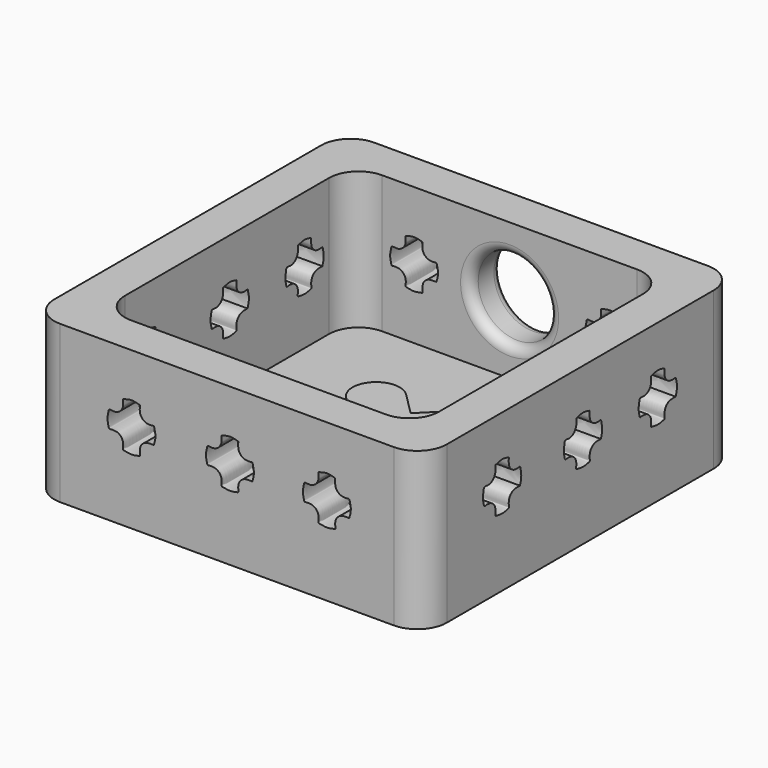
from build123d import *

# Parameters (mm, degrees)
F1_DEPTH      = 2
F2_W          = 40
F2_H          = 40
F3_DEPTH      = 2
F3_DEPTH_BACK = 14
F4_DEPTH      = 2
F5_R          = 3
F6_R          = 4
F7_DEPTH      = 25
F8_R          = 1
F10_DEPTH     = 25
F12_DEPTH     = 45.8


# Not quite as in the source:
# - a pattern or mirror of a feature is missing from the dataset's text; its kind, count and spacing are read off the source's solid


with BuildPart() as f1:
    # F0 (on Top) → F1 (new body)
    with BuildSketch(Plane.XY):
        with BuildLine():
            Line((4, -0.6058874503), (1.6970562748, 1.6970562748))
            ThreePointArc((1.6970562748, 1.6970562748), (-1.6970562748, 1.6970562748), (-1.6970562748, -1.6970562748))
            Line((-1.6970562748, -1.6970562748), (0.6058874503, -4))
            Line((0.6058874503, -4), (-1.6970562748, -6.3029437252))
            ThreePointArc((-1.6970562748, -6.3029437252), (-1.6970562748, -9.6970562748), (1.6970562748, -9.6970562748))
            Line((1.6970562748, -9.6970562748), (4, -7.3941125497))
            Line((4, -7.3941125497), (6.3029437252, -9.6970562748))
            ThreePointArc((6.3029437252, -9.6970562748), (9.6970562748, -9.6970562748), (9.6970562748, -6.3029437252))
            Line((9.6970562748, -6.3029437252), (7.3941125497, -4))
            Line((7.3941125497, -4), (9.6970562748, -1.6970562748))
            ThreePointArc((9.6970562748, -1.6970562748), (9.6970562748, 1.6970562748), (6.3029437252, 1.6970562748))
            Line((6.3029437252, 1.6970562748), (4, -0.6058874503))
        make_face()
    extrude(amount=F1_DEPTH)

    # F2 (on Top) → F4 (join)
    with BuildSketch(Plane.XY):
        with BuildLine():
            Line((17, 12), (-9, 12))
            ThreePointArc((-9, 12), (-11.1213203436, 11.1213203436), (-12, 9))
            Line((-12, 9), (-12, -17))
            ThreePointArc((-12, -17), (-11.1213203436, -19.1213203436), (-9, -20))
            Line((-9, -20), (17, -20))
            ThreePointArc((17, -20), (19.1213203436, -19.1213203436), (20, -17))
            Line((20, -17), (20, 9))
            ThreePointArc((20, 9), (19.1213203436, 11.1213203436), (17, 12))
        make_face()
    extrude(amount=-F4_DEPTH)


with BuildPart() as f3:
    # F2 (on Top) → F3 (new body, two sides)
    with BuildSketch(Plane.XY) as f3_sk:
        with Locations((4, -4)):
            Rectangle(F2_W, F2_H)
        with BuildLine():
            ThreePointArc((-12, 9), (-11.1213203436, 11.1213203436), (-9, 12))
            Line((-9, 12), (17, 12))
            ThreePointArc((17, 12), (19.1213203436, 11.1213203436), (20, 9))
            Line((20, 9), (20, -17))
            ThreePointArc((20, -17), (19.1213203436, -19.1213203436), (17, -20))
            Line((17, -20), (-9, -20))
            ThreePointArc((-9, -20), (-11.1213203436, -19.1213203436), (-12, -17))
            Line((-12, -17), (-12, 9))
        make_face(mode=Mode.SUBTRACT)
    extrude(amount=-F3_DEPTH)
    extrude(f3_sk.sketch, amount=F3_DEPTH_BACK)

    # F5
    f5_edges = [f3.edges().sort_by_distance(p)[0] for p in [
        (-16, -24, 6),
        (-16, 16, 6),
        (24, 16, 6),
        (24, -24, 6),
    ]]
    fillet(f5_edges, radius=F5_R)

    # F6 (on face) → F7 (cut)
    with BuildSketch(Plane(origin=(0, 16, 0), x_dir=(-1, 0, 0), z_dir=(0, 1, 0))):
        with Locations((-4, 7)):
            Circle(F6_R)
    extrude(amount=-F7_DEPTH, mode=Mode.SUBTRACT)

    # F8
    f8_edges = [f3.edges().sort_by_distance(p)[0] for p in [
        (8, 16, 7),
        (8, 12, 7),
    ]]
    fillet(f8_edges, radius=F8_R)

    # F9 (on face) → F10 (cut)
    with BuildSketch(Plane.XZ.offset(24)):
        with BuildLine():
            add(Edge.make_bspline(
                [(-6.5840265518, 9.3437267381), (-6.286408434, 9.4275877117), (-5.7023076012, 9.5950066295), (-5.1532978898, 9.4254739497), (-4.8840257185, 9.3437267381)],
                knots=[0, 0, 0, 0, 0.5095712537, 1, 1, 1, 1], degree=3))
            add(Edge.make_bspline(
                [(-6.5840265518, 9.3437267381), (-6.5841696509, 9.2446224959), (-6.5844438767, 9.0547054322), (-6.5825932662, 8.7979336724), (-6.5988182275, 8.609172852), (-6.7707458313, 8.2509387062), (-6.9735726246, 8.079923012), (-7.250701533, 7.9446481243), (-7.5437717101, 7.8925599497), (-8.077660269, 8.0248628406), (-8.0810784131, 7.6236458981), (-8.1649065579, 7.3625472686), (-8.1781814391, 7.0265606699), (-8.1535417531, 6.7364119598), (-8.0802507294, 6.4930721252), (-8.0454514039, 6.1628262916), (-7.7981073276, 6.2405421407), (-7.4978512443, 6.2260779569), (-7.2459325913, 6.194091152), (-7.0561037114, 6.118114005), (-6.8276872429, 5.9377813233), (-6.7252267328, 5.7961916646), (-6.6269718231, 5.6163632202), (-6.5808026719, 5.3578690355), (-6.5679532623, 5.1331167152), (-6.6600281407, 4.7409543997), (-6.3080518593, 4.7336285908), (-5.9846905263, 4.6481815982), (-5.698126367, 4.6467208848), (-5.4347625835, 4.6517875366), (-5.0847116703, 4.7519672139), (-4.8238785102, 4.7525241561), (-4.8965607786, 5.139699186), (-4.8941701444, 5.3873990167), (-4.7921945694, 5.737853877), (-4.6502771673, 5.9263389013), (-4.3801585127, 6.1591111569), (-3.953865455, 6.2407381261), (-3.6306534992, 6.2287716349), (-3.4628957185, 6.222560627)],
                knots=[0, 0, 0, 0, 0.0273605905, 0.0524320947, 0.0745076412, 0.1056108167, 0.1318649214, 0.158948127, 0.1874687016, 0.220995097, 0.2482860623, 0.2755720453, 0.3045111481, 0.3315301836, 0.3578655515, 0.3837385363, 0.4059679792, 0.434252013, 0.4594532962, 0.4822711791, 0.5090972104, 0.530231005, 0.5527300135, 0.5781274322, 0.6031996615, 0.6315546276, 0.6576667534, 0.6876672756, 0.714256594, 0.7402463844, 0.7710533559, 0.7932728015, 0.8216277676, 0.8482190477, 0.8777914221, 0.9023565188, 0.9315770045, 0.9644861842, 1, 1, 1, 1], degree=3))
            add(Edge.make_bspline(
                [(-4.8840257185, 9.3437267381), (-4.8935755093, 9.1506042586), (-4.9112536502, 8.7832152223), (-4.7756004039, 8.3288680656), (-4.4316068524, 8.0186270395), (-4.0888222693, 7.9133263313), (-3.6792961769, 7.9039789989), (-3.4252992175, 7.9777305663), (-3.3873804743, 7.6560080441), (-3.2915965783, 7.2992742436), (-3.2932886729, 6.9532412937), (-3.3298571311, 6.6299537163), (-3.4169636222, 6.3649352611), (-3.4628957185, 6.222560627)],
                knots=[0, 0, 0, 0, 0.1117445823, 0.2125923647, 0.3107430927, 0.4000660841, 0.4960442665, 0.5626441507, 0.6379036869, 0.7311412958, 0.8178947498, 0.9022950941, 1, 1, 1, 1], degree=3))
        make_face()
        with BuildLine():
            add(Edge.make_bspline(
                [(3.4491739476, 9.3437267381), (3.7467920654, 9.4275877117), (4.3308928982, 9.5950066295), (4.8799026096, 9.4254739497), (5.1491747809, 9.3437267381)],
                knots=[0, 0, 0, 0, 0.5095712537, 1, 1, 1, 1], degree=3))
            add(Edge.make_bspline(
                [(3.4491739476, 9.3437267381), (3.4490308485, 9.2446224959), (3.4487566227, 9.0547054322), (3.4506072332, 8.7979336724), (3.4343822719, 8.609172852), (3.2624546681, 8.2509387062), (3.0596278748, 8.079923012), (2.7824989664, 7.9446481243), (2.4894287893, 7.8925599497), (1.9555402304, 8.0248628406), (1.9521220863, 7.6236458981), (1.8682939415, 7.3625472686), (1.8550190603, 7.0265606699), (1.8796587463, 6.7364119598), (1.95294977, 6.4930721252), (1.9877490955, 6.1628262916), (2.2350931718, 6.2405421407), (2.5353492551, 6.2260779569), (2.7872679081, 6.194091152), (2.977096788, 6.118114005), (3.2055132565, 5.9377813233), (3.3079737666, 5.7961916646), (3.4062286763, 5.6163632202), (3.4523978275, 5.3578690355), (3.4652472371, 5.1331167152), (3.3731723587, 4.7409543997), (3.7251486401, 4.7336285908), (4.0485099731, 4.6481815982), (4.3350741324, 4.6467208848), (4.5984379159, 4.6517875366), (4.9484888291, 4.7519672139), (5.2093219892, 4.7525241561), (5.1366397208, 5.139699186), (5.139030355, 5.3873990167), (5.24100593, 5.737853877), (5.3829233321, 5.9263389013), (5.6530419867, 6.1591111569), (6.0793350444, 6.2407381261), (6.4025470002, 6.2287716349), (6.5703047809, 6.222560627)],
                knots=[0, 0, 0, 0, 0.0273605905, 0.0524320947, 0.0745076412, 0.1056108167, 0.1318649214, 0.158948127, 0.1874687016, 0.220995097, 0.2482860623, 0.2755720453, 0.3045111481, 0.3315301836, 0.3578655515, 0.3837385363, 0.4059679792, 0.434252013, 0.4594532962, 0.4822711791, 0.5090972104, 0.530231005, 0.5527300135, 0.5781274322, 0.6031996615, 0.6315546276, 0.6576667534, 0.6876672756, 0.714256594, 0.7402463844, 0.7710533559, 0.7932728015, 0.8216277676, 0.8482190477, 0.8777914221, 0.9023565188, 0.9315770045, 0.9644861842, 1, 1, 1, 1], degree=3))
            add(Edge.make_bspline(
                [(5.1491747809, 9.3437267381), (5.1396249901, 9.1506042586), (5.1219468492, 8.7832152223), (5.2576000955, 8.3288680656), (5.601593647, 8.0186270395), (5.9443782301, 7.9133263313), (6.3539043225, 7.9039789989), (6.6079012819, 7.9777305663), (6.6458200251, 7.6560080441), (6.7416039211, 7.2992742436), (6.7399118265, 6.9532412937), (6.7033433683, 6.6299537163), (6.6162368772, 6.3649352611), (6.5703047809, 6.222560627)],
                knots=[0, 0, 0, 0, 0.1117445823, 0.2125923647, 0.3107430927, 0.4000660841, 0.4960442665, 0.5626441507, 0.6379036869, 0.7311412958, 0.8178947498, 0.9022950941, 1, 1, 1, 1], degree=3))
        make_face()
        with BuildLine():
            add(Edge.make_bspline(
                [(13.3281609331, 9.2647962186), (13.625779051, 9.3486571921), (14.2098798838, 9.5160761099), (14.7588895952, 9.3465434302), (15.0281617664, 9.2647962186)],
                knots=[0, 0, 0, 0, 0.5095712537, 1, 1, 1, 1], degree=3))
            add(Edge.make_bspline(
                [(13.3281609331, 9.2647962186), (13.3280178341, 9.1656919763), (13.3277436082, 8.9757749126), (13.3295942187, 8.7190031529), (13.3133692574, 8.5302423325), (13.1414416536, 8.1720081867), (12.9386148603, 8.0009924924), (12.6614859519, 7.8657176048), (12.3684157749, 7.8136294302), (11.834527216, 7.9459323211), (11.8311090719, 7.5447153785), (11.7472809271, 7.2836167491), (11.7340060459, 6.9476301504), (11.7586457319, 6.6574814402), (11.8319367556, 6.4141416057), (11.866736081, 6.0838957721), (12.1140801574, 6.1616116212), (12.4143362407, 6.1471474374), (12.6662548936, 6.1151606325), (12.8560837735, 6.0391834855), (13.084500242, 5.8588508038), (13.1869607522, 5.7172611451), (13.2852156618, 5.5374327007), (13.3313848131, 5.278938516), (13.3442342227, 5.0541861957), (13.2521593443, 4.6620238801), (13.6041356256, 4.6546980712), (13.9274969586, 4.5692510786), (14.2140611179, 4.5677903652), (14.4774249014, 4.5728570171), (14.8274758147, 4.6730366943), (15.0883089747, 4.6735936366), (15.0156267064, 5.0607686665), (15.0180173406, 5.3084684972), (15.1199929156, 5.6589233574), (15.2619103177, 5.8474083818), (15.5320289723, 6.0801806374), (15.9583220299, 6.1618076066), (16.2815339858, 6.1498411154), (16.4492917664, 6.1436301075)],
                knots=[0, 0, 0, 0, 0.0273605905, 0.0524320947, 0.0745076412, 0.1056108167, 0.1318649214, 0.158948127, 0.1874687016, 0.220995097, 0.2482860623, 0.2755720453, 0.3045111481, 0.3315301836, 0.3578655515, 0.3837385363, 0.4059679792, 0.434252013, 0.4594532962, 0.4822711791, 0.5090972104, 0.530231005, 0.5527300135, 0.5781274322, 0.6031996615, 0.6315546276, 0.6576667534, 0.6876672756, 0.714256594, 0.7402463844, 0.7710533559, 0.7932728015, 0.8216277676, 0.8482190477, 0.8777914221, 0.9023565188, 0.9315770045, 0.9644861842, 1, 1, 1, 1], degree=3))
            add(Edge.make_bspline(
                [(15.0281617664, 9.2647962186), (15.0186119756, 9.0716737391), (15.0009338347, 8.7042847028), (15.1365870811, 8.2499375461), (15.4805806325, 7.93969652), (15.8233652156, 7.8343958117), (16.232891308, 7.8250484794), (16.4868882675, 7.8988000468), (16.5248070106, 7.5770775246), (16.6205909067, 7.2203437241), (16.618898812, 6.8743107742), (16.5823303539, 6.5510231967), (16.4952238628, 6.2860047416), (16.4492917664, 6.1436301075)],
                knots=[0, 0, 0, 0, 0.1117445823, 0.2125923647, 0.3107430927, 0.4000660841, 0.4960442665, 0.5626441507, 0.6379036869, 0.7311412958, 0.8178947498, 0.9022950941, 1, 1, 1, 1], degree=3))
        make_face()
    f10 = extrude(amount=-F10_DEPTH, mode=Mode.SUBTRACT)

    # F10_copies: F10 across plane
    add(f10.mirror(Plane.ZX.offset(-4)), mode=Mode.SUBTRACT)

    # F11 (on face) → F12 (cut)
    with BuildSketch(Plane.YZ.offset(24)):
        with BuildLine():
            add(Edge.make_bspline(
                [(-14.8045055538, 9.6274732526), (-14.5068874359, 9.7113342261), (-13.9227866031, 9.8787531439), (-13.3737768917, 9.7092204642), (-13.1045047205, 9.6274732526)],
                knots=[0, 0, 0, 0, 0.5095712537, 1, 1, 1, 1], degree=3))
            add(Edge.make_bspline(
                [(-14.8045055538, 9.6274732526), (-14.8046486528, 9.5283690103), (-14.8049228787, 9.3384519466), (-14.8030722682, 9.0816801869), (-14.8192972295, 8.8929193665), (-14.9912248333, 8.5346852207), (-15.1940516266, 8.3636695264), (-15.471180535, 8.2283946388), (-15.764250712, 8.1763064642), (-16.2981392709, 8.3086093551), (-16.301557415, 7.9073924125), (-16.3853855598, 7.6462937831), (-16.398660441, 7.3103071844), (-16.374020755, 7.0201584742), (-16.3007297313, 6.7768186396), (-16.2659304059, 6.4465728061), (-16.0185863295, 6.5242886552), (-15.7183302462, 6.5098244713), (-15.4664115933, 6.4778376665), (-15.2765827134, 6.4018605195), (-15.0481662449, 6.2215278378), (-14.9457057347, 6.0799381791), (-14.8474508251, 5.9001097346), (-14.8012816738, 5.64161555), (-14.7884322642, 5.4168632296), (-14.8805071426, 5.0247009141), (-14.5285308613, 5.0173751052), (-14.2051695283, 4.9319281126), (-13.918605369, 4.9304673992), (-13.6552415854, 4.9355340511), (-13.3051906722, 5.0357137283), (-13.0443575122, 5.0362706705), (-13.1170397805, 5.4234457005), (-13.1146491463, 5.6711455312), (-13.0126735713, 6.0216003914), (-12.8707561692, 6.2100854158), (-12.6006375146, 6.4428576714), (-12.174344457, 6.5244846406), (-11.8511325011, 6.5125181494), (-11.6833747205, 6.5063071415)],
                knots=[0, 0, 0, 0, 0.0273605905, 0.0524320947, 0.0745076412, 0.1056108167, 0.1318649214, 0.158948127, 0.1874687016, 0.220995097, 0.2482860623, 0.2755720453, 0.3045111481, 0.3315301836, 0.3578655515, 0.3837385363, 0.4059679792, 0.434252013, 0.4594532962, 0.4822711791, 0.5090972104, 0.530231005, 0.5527300135, 0.5781274322, 0.6031996615, 0.6315546276, 0.6576667534, 0.6876672756, 0.714256594, 0.7402463844, 0.7710533559, 0.7932728015, 0.8216277676, 0.8482190477, 0.8777914221, 0.9023565188, 0.9315770045, 0.9644861842, 1, 1, 1, 1], degree=3))
            add(Edge.make_bspline(
                [(-13.1045047205, 9.6274732526), (-13.1140545113, 9.4343507731), (-13.1317326522, 9.0669617368), (-12.9960794058, 8.6126145801), (-12.6520858544, 8.302373554), (-12.3093012713, 8.1970728457), (-11.8997751789, 8.1877255134), (-11.6457782194, 8.2614770808), (-11.6078594763, 7.9397545586), (-11.5120755802, 7.5830207581), (-11.5137676749, 7.2369878082), (-11.550336133, 6.9137002307), (-11.6374426241, 6.6486817756), (-11.6833747205, 6.5063071415)],
                knots=[0, 0, 0, 0, 0.1117445823, 0.2125923647, 0.3107430927, 0.4000660841, 0.4960442665, 0.5626441507, 0.6379036869, 0.7311412958, 0.8178947498, 0.9022950941, 1, 1, 1, 1], degree=3))
        make_face()
        with BuildLine():
            add(Edge.make_bspline(
                [(-4.5020328835, 9.6274732526), (-4.2044147656, 9.7113342261), (-3.6203139328, 9.8787531439), (-3.0713042214, 9.7092204642), (-2.8020320501, 9.6274732526)],
                knots=[0, 0, 0, 0, 0.5095712537, 1, 1, 1, 1], degree=3))
            add(Edge.make_bspline(
                [(-4.5020328835, 9.6274732526), (-4.5021759825, 9.5283690103), (-4.5024502083, 9.3384519466), (-4.5005995979, 9.0816801869), (-4.5168245592, 8.8929193665), (-4.6887521629, 8.5346852207), (-4.8915789562, 8.3636695264), (-5.1687078647, 8.2283946388), (-5.4617780417, 8.1763064642), (-5.9956666006, 8.3086093551), (-5.9990847447, 7.9073924125), (-6.0829128895, 7.6462937831), (-6.0961877707, 7.3103071844), (-6.0715480847, 7.0201584742), (-5.998257061, 6.7768186396), (-5.9634577355, 6.4465728061), (-5.7161136592, 6.5242886552), (-5.4158575759, 6.5098244713), (-5.163938923, 6.4778376665), (-4.9741100431, 6.4018605195), (-4.7456935746, 6.2215278378), (-4.6432330644, 6.0799381791), (-4.5449781547, 5.9001097346), (-4.4988090035, 5.64161555), (-4.4859595939, 5.4168632296), (-4.5780344723, 5.0247009141), (-4.2260581909, 5.0173751052), (-3.902696858, 4.9319281126), (-3.6161326986, 4.9304673992), (-3.3527689151, 4.9355340511), (-3.0027180019, 5.0357137283), (-2.7418848418, 5.0362706705), (-2.8145671102, 5.4234457005), (-2.812176476, 5.6711455312), (-2.710200901, 6.0216003914), (-2.5682834989, 6.2100854158), (-2.2981648443, 6.4428576714), (-1.8718717866, 6.5244846406), (-1.5486598308, 6.5125181494), (-1.3809020501, 6.5063071415)],
                knots=[0, 0, 0, 0, 0.0273605905, 0.0524320947, 0.0745076412, 0.1056108167, 0.1318649214, 0.158948127, 0.1874687016, 0.220995097, 0.2482860623, 0.2755720453, 0.3045111481, 0.3315301836, 0.3578655515, 0.3837385363, 0.4059679792, 0.434252013, 0.4594532962, 0.4822711791, 0.5090972104, 0.530231005, 0.5527300135, 0.5781274322, 0.6031996615, 0.6315546276, 0.6576667534, 0.6876672756, 0.714256594, 0.7402463844, 0.7710533559, 0.7932728015, 0.8216277676, 0.8482190477, 0.8777914221, 0.9023565188, 0.9315770045, 0.9644861842, 1, 1, 1, 1], degree=3))
            add(Edge.make_bspline(
                [(-2.8020320501, 9.6274732526), (-2.811581841, 9.4343507731), (-2.8292599818, 9.0669617368), (-2.6936067355, 8.6126145801), (-2.3496131841, 8.302373554), (-2.0068286009, 8.1970728457), (-1.5973025085, 8.1877255134), (-1.3433055491, 8.2614770808), (-1.3053868059, 7.9397545586), (-1.2096029099, 7.5830207581), (-1.2112950046, 7.2369878082), (-1.2478634627, 6.9137002307), (-1.3349699538, 6.6486817756), (-1.3809020501, 6.5063071415)],
                knots=[0, 0, 0, 0, 0.1117445823, 0.2125923647, 0.3107430927, 0.4000660841, 0.4960442665, 0.5626441507, 0.6379036869, 0.7311412958, 0.8178947498, 0.9022950941, 1, 1, 1, 1], degree=3))
        make_face()
        with BuildLine():
            add(Edge.make_bspline(
                [(5.0289737992, 9.548542733), (5.3265919171, 9.6324037066), (5.9106927499, 9.7998226244), (6.4597024613, 9.6302899447), (6.7289746325, 9.548542733)],
                knots=[0, 0, 0, 0, 0.5095712537, 1, 1, 1, 1], degree=3))
            add(Edge.make_bspline(
                [(5.0289737992, 9.548542733), (5.0288307002, 9.4494384908), (5.0285564743, 9.2595214271), (5.0304070848, 9.0027496673), (5.0141821235, 8.813988847), (4.8422545197, 8.4557547012), (4.6394277264, 8.2847390069), (4.362298818, 8.1494641193), (4.069228641, 8.0973759447), (3.5353400821, 8.2296788356), (3.531921938, 7.828461893), (3.4480937932, 7.5673632636), (3.4348189119, 7.2313766649), (3.459458598, 6.9412279547), (3.5327496217, 6.6978881201), (3.5675489471, 6.3676422866), (3.8148930235, 6.4453581356), (4.1151491068, 6.4308939518), (4.3670677597, 6.398907147), (4.5568966396, 6.3229299999), (4.7853131081, 6.1425973183), (4.8877736183, 6.0010076596), (4.9860285279, 5.8211792151), (5.0321976791, 5.5626850305), (5.0450470888, 5.3379327101), (4.9529722104, 4.9457703946), (5.3049484917, 4.9384445857), (5.6283098247, 4.8529975931), (5.914873984, 4.8515368797), (6.1782377675, 4.8566035315), (6.5282886808, 4.9567832088), (6.7891218408, 4.957340151), (6.7164395725, 5.344515181), (6.7188302066, 5.5922150117), (6.8208057816, 5.9426698719), (6.9627231837, 6.1311548963), (7.2328418384, 6.3639271518), (7.659134896, 6.4455541211), (7.9823468519, 6.4335876298), (8.1501046325, 6.4273766219)],
                knots=[0, 0, 0, 0, 0.0273605905, 0.0524320947, 0.0745076412, 0.1056108167, 0.1318649214, 0.158948127, 0.1874687016, 0.220995097, 0.2482860623, 0.2755720453, 0.3045111481, 0.3315301836, 0.3578655515, 0.3837385363, 0.4059679792, 0.434252013, 0.4594532962, 0.4822711791, 0.5090972104, 0.530231005, 0.5527300135, 0.5781274322, 0.6031996615, 0.6315546276, 0.6576667534, 0.6876672756, 0.714256594, 0.7402463844, 0.7710533559, 0.7932728015, 0.8216277676, 0.8482190477, 0.8777914221, 0.9023565188, 0.9315770045, 0.9644861842, 1, 1, 1, 1], degree=3))
            add(Edge.make_bspline(
                [(6.7289746325, 9.548542733), (6.7194248417, 9.3554202536), (6.7017467008, 8.9880312173), (6.8373999472, 8.5336840605), (7.1813934986, 8.2234430345), (7.5241780817, 8.1181423262), (7.9337041741, 8.1087949939), (8.1877011336, 8.1825465612), (8.2256198767, 7.8608240391), (8.3214037728, 7.5040902386), (8.3197116781, 7.1580572887), (8.28314322, 6.8347697112), (8.1960367288, 6.5697512561), (8.1501046325, 6.4273766219)],
                knots=[0, 0, 0, 0, 0.1117445823, 0.2125923647, 0.3107430927, 0.4000660841, 0.4960442665, 0.5626441507, 0.6379036869, 0.7311412958, 0.8178947498, 0.9022950941, 1, 1, 1, 1], degree=3))
        make_face()
    extrude(amount=-F12_DEPTH, mode=Mode.SUBTRACT)


solid = Compound([f1.part, f3.part])
